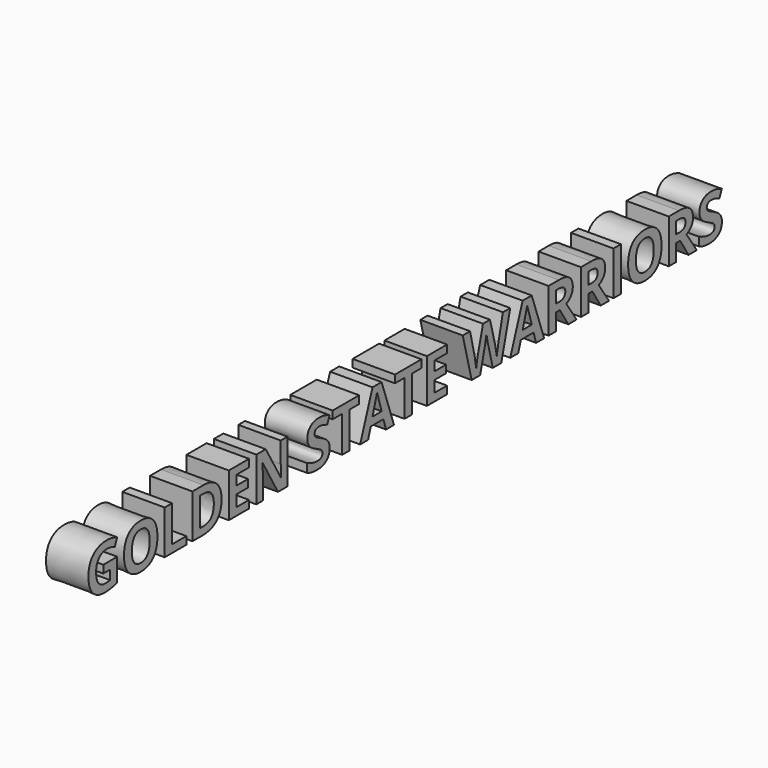
from build123d import *

# Parameters (mm, degrees)
F0_TEXT_SIZE = 367.8288724687
F1_DEPTH     = 254


# Not quite as in the source:
# - Text() gives the source's letters only with a copy of the font that has no kerning and outlines rounded to 1/6400 em; it was checked with that copy


with BuildPart() as f1:
    # F0 (on Right) → F1 (new body)
    with BuildSketch(Plane.YZ):
        with Locations((-333.3254158497, 0)):
            Text('GOLDEN STATE WARRIORS', F0_TEXT_SIZE, font='Open Sans', font_style=FontStyle.BOLD, text_align=(TextAlign.LEFT, TextAlign.BOTTOM))
    extrude(amount=F1_DEPTH)


solid = f1.part
